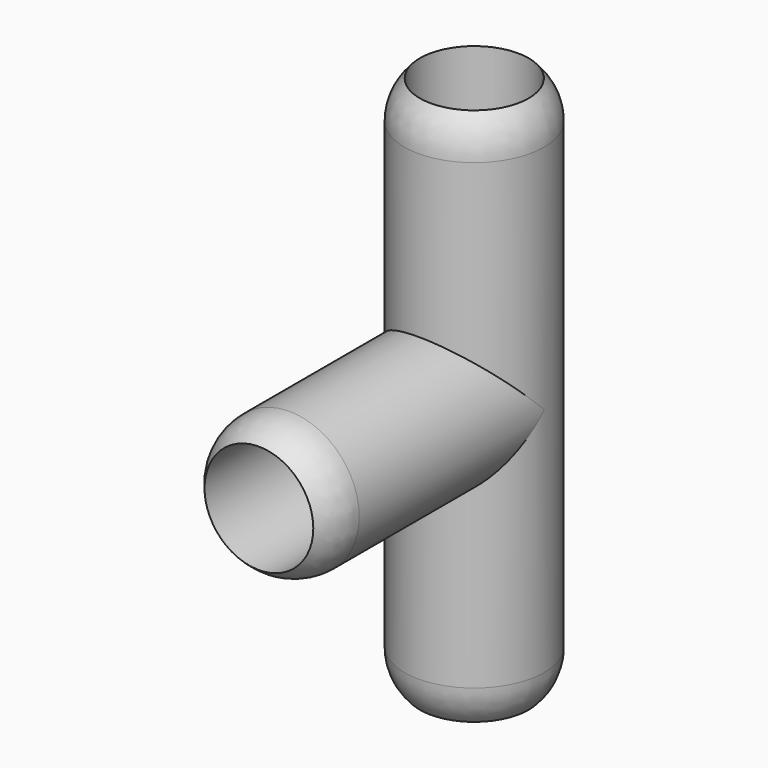
from build123d import *

# Parameters (mm, degrees)
F0_R     = 6.5
F0_R_2   = 5.05
F1_DEPTH = 25
F2_DEPTH = 25
F3_R     = 6.5
F3_R_2   = 5.05
F4_DEPTH = 25


# Not quite as in the source:
# - a fillet or chamfer that OpenCascade refuses, or shapes differently, is made with other operations: its cross-section is extruded or revolved along the edge and cut away or added


with BuildPart() as f1:
    # F0 (on Top) → F1 (new body)
    with BuildSketch(Plane.XY):
        Circle(F0_R)
        Circle(F0_R_2, mode=Mode.SUBTRACT)
    extrude(amount=F1_DEPTH)

    # F0 (on Top) → F2 (join)
    with BuildSketch(Plane.XY):
        Circle(F0_R)
        Circle(F0_R_2, mode=Mode.SUBTRACT)
    extrude(amount=-F2_DEPTH)

    # F3 (on Front) → F4 (join)
    with BuildSketch(Plane.XZ):
        Circle(F3_R)
        Circle(F3_R_2, mode=Mode.SUBTRACT)
    extrude(amount=F4_DEPTH)

    # F5: fillet of radius 5 on 3 edges, made by hand

    # F5_s1 → F5_t2 (revolve, cut)
    with BuildSketch(Plane.XY):
        with BuildLine():
            ThreePointArc((6.5, -21.4789916217), (6.1233105022, -23.3829348982), (5.05, -25))
            Line((5.05, -25), (6.5, -25))
            Line((6.5, -25), (6.5, -21.4789916217))
        make_face()
    revolve(axis=Axis((0, -25, 0), (0, -1, 0)), mode=Mode.SUBTRACT)

    # F5_s3 → F5_t4 (revolve, cut)
    with BuildSketch(Plane.XZ):
        with BuildLine():
            ThreePointArc((6.5, -21.4789916217), (6.1233105022, -23.3829348982), (5.05, -25))
            Line((5.05, -25), (6.5, -25))
            Line((6.5, -25), (6.5, -21.4789916217))
        make_face()
    revolve(axis=Axis((0, 0, -25), (0, 0, 1)), mode=Mode.SUBTRACT)

    # F5_s5 → F5_t6 (revolve, cut)
    with BuildSketch(Plane.XZ):
        with BuildLine():
            ThreePointArc((6.5, 21.4789916217), (6.1233105022, 23.3829348982), (5.05, 25))
            Line((5.05, 25), (6.5, 25))
            Line((6.5, 25), (6.5, 21.4789916217))
        make_face()
    revolve(axis=Axis((0, 0, 25), (0, 0, 1)), mode=Mode.SUBTRACT)


solid = f1.part
